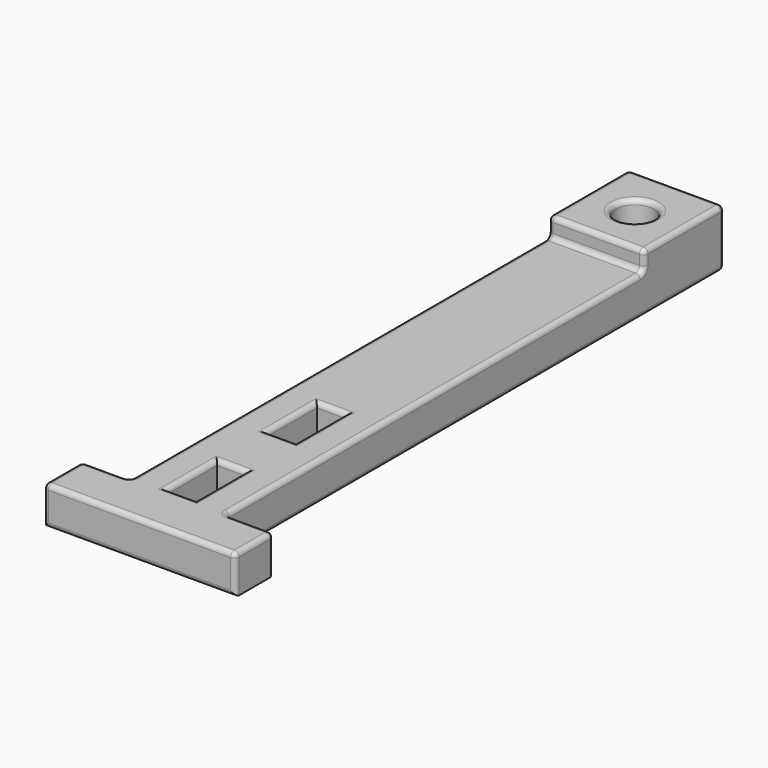
from build123d import *

# Parameters (mm, degrees)
F0_W     = 20
F0_H     = 130
F0_W_2   = 6
F0_H_2   = 13
F0_H_3   = 10
F0_W_3   = 10
F1_DEPTH = 8
F2_R     = 4
F3_DEPTH = 50
F2_W     = 20
F2_H     = 20.9063310176
F4_DEPTH = 4
F5_F1_R  = 1
F5_F2_R  = 1


with BuildPart() as f1:
    # F0 (on Top) → F1 (new body)
    with BuildSketch(Plane.XY):
        with Locations((-46.5529351234, 65.628703773)):
            Rectangle(F0_W, F0_H)
        with Locations((-46.5529351234, 8.128703773)):
            Rectangle(F0_W_2, F0_H_2, mode=Mode.SUBTRACT)
        with Locations((-46.5529351234, 34.128703773)):
            Rectangle(F0_W_2, F0_H_2, mode=Mode.SUBTRACT)
        with Locations((-46.5529351234, -4.371296227)):
            Rectangle(F0_W, F0_H_3)
        with Locations((-61.5529351234, -4.371296227)):
            Rectangle(F0_W_3, F0_H_3)
        with Locations((-31.5529351234, -4.371296227)):
            Rectangle(F0_W_3, F0_H_3)
    extrude(amount=F1_DEPTH)

    # F2 (on face) → F3 (cut, symmetric)
    with BuildSketch(Plane.XY.offset(8)):
        with Locations((-46.5529351234, 119.7651425898)):
            Circle(F2_R)
    extrude(amount=F3_DEPTH, both=True, mode=Mode.SUBTRACT)

    # F2 (on face) → F4 (join)
    with BuildSketch(Plane.XY.offset(8)):
        with Locations((-46.5529351234, 120.1755382642)):
            Rectangle(F2_W, F2_H)
        with Locations((-46.5529351234, 119.7651425898)):
            Circle(F2_R, mode=Mode.SUBTRACT)
    extrude(amount=F4_DEPTH)

    # F5: fillet of radius 1 on 35 edges, made by hand

    # F5_f1
    f5_f1_edges = [f1.edges().sort_by_distance(p)[0] for p in [
        (-46.5529351234, 109.7223727554, 8),
        (-36.5529351234, 0.628703773, 4),
        (-56.5529351234, 0.628703773, 4),
    ]]
    fillet(f5_f1_edges, radius=F5_F1_R)

    # F5_f2
    f5_f2_edges = [f1.edges().sort_by_distance(p)[0] for p in [
        (-36.5529351234, 55.1755382642, 8),
        (-31.0529351234, 0.628703773, 8),
        (-26.5529351234, -4.371296227, 8),
        (-46.5529351234, -9.371296227, 8),
        (-66.5529351234, -4.371296227, 8),
        (-62.0529351234, 0.628703773, 8),
        (-56.5529351234, 55.1755382642, 8),
        (-49.5529351234, 8.128703773, 8),
        (-46.5529351234, 1.628703773, 8),
        (-46.5529351234, 14.628703773, 8),
        (-43.5529351234, 8.128703773, 8),
        (-46.5529351234, 40.628703773, 8),
        (-49.5529351234, 34.128703773, 8),
        (-43.5529351234, 34.128703773, 8),
        (-46.5529351234, 27.628703773, 8),
        (-36.5529351234, 66.128703773, 0),
        (-56.5529351234, 66.128703773, 0),
        (-46.5529351234, 130.628703773, 12),
        (-56.5529351234, 120.1755382642, 12),
        (-46.5529351234, 109.7223727554, 12),
        (-36.5529351234, 120.1755382642, 12),
        (-50.5529351234, 119.7651425898, 12),
        (-26.5529351234, 0.628703773, 4),
        (-31.0529351234, 0.628703773, 0),
        (-66.5529351234, 0.628703773, 4),
        (-62.0529351234, 0.628703773, 0),
        (-36.5529351234, 130.628703773, 6),
        (-56.5529351234, 130.628703773, 6),
        (-46.5529351234, 130.628703773, 0),
        (-66.5529351234, -9.371296227, 4),
        (-26.5529351234, -9.371296227, 4),
        (-46.5529351234, -9.371296227, 0),
        (-56.8458283423, 0.9215969918, 0),
        (-36.2600419046, 0.9215969918, 0),
        (-56.5529351234, 109.4294795366, 8.2928932188),
        (-56.8458283423, 0.9215969918, 8),
        (-36.2600419046, 0.9215969918, 8),
        (-36.5529351234, 109.4294795366, 8.2928932188),
    ]]
    fillet(f5_f2_edges, radius=F5_F2_R)


solid = f1.part
